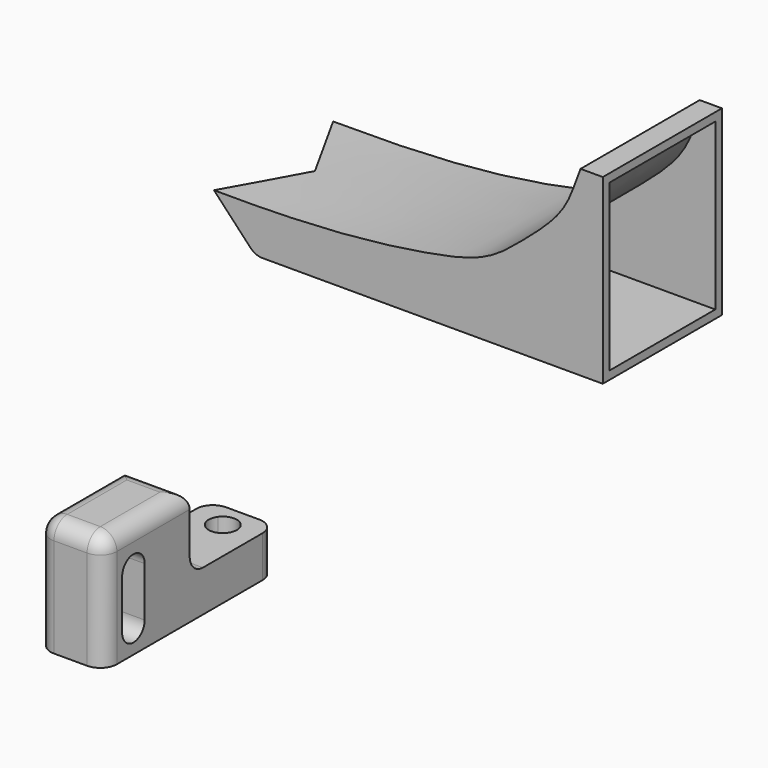
from build123d import *

# Parameters (mm, degrees)
F0_W      = 47
F0_H      = 18
F1_DEPTH  = 22
F4_DEPTH  = 25
F5_DEPTH  = 25
F7_T      = -1
F2_W      = 16
F2_H      = 20
F8_DEPTH  = 1
F9_W      = 8
F9_H      = 26
F10_DEPTH = 14
F11_W     = 13
F11_H     = 9
F12_DEPTH = 25
F13_R     = 2
F15_DEPTH = 25
F17_DEPTH = 25
F19_W     = 6.1407467425
F19_H     = 16
F20_DEPTH = 2
F21_R     = 2
F23_DEPTH = 16
F24_DEPTH = 25


# Not quite as in the source:
# - ends of sketch curves that miss each other by under 0.0002 mm in the source are joined


with BuildPart() as f1:
    # F0 (on Top) → F1 (new body)
    with BuildSketch(Plane.XY):
        with Locations((-23.5, 9)):
            Rectangle(F0_W, F0_H)
    extrude(amount=F1_DEPTH)

    # F3 (on face) → F4 (cut)
    with BuildSketch(Plane.XZ):
        with BuildLine():
            add(Edge.make_bspline(
                [(-2.6882688196, 22), (-3.2770454434, 20.6391466758), (-4.1784598757, 16.8748983141), (-9.4041486141, 12.3630724805), (-13.9335501605, 8.4565637973), (-23.0360767099, 6.5368633633), (-34.0870933489, 5.200595818), (-47, 5.3147859871)],
                knots=[0, 0, 0, 0, 0.1494824851, 0.3218138719, 0.4814084184, 0.6655862643, 1, 1, 1, 1], degree=3))
            Line((-2.6882688196, 22), (-47, 22))
            Line((-47, 22), (-47, 5.3147859871))
        make_face()
    extrude(amount=-F4_DEPTH, mode=Mode.SUBTRACT)

    # F3 (on face) → F5 (cut)
    with BuildSketch(Plane.XZ):
        Polygon((-42, 0), (-47, 5.3147859871), (-47, 0), align=None)
    extrude(amount=-F5_DEPTH, mode=Mode.SUBTRACT)

    # F7
    f7_openings = [f1.faces().sort_by_distance(p)[0] for p in [
        (-44.5, 9, 2.657393),
    ]]
    offset(amount=F7_T, openings=f7_openings, kind=Kind.INTERSECTION)

    # F2 (on face) → F8 (cut)
    with BuildSketch(Plane.YZ):
        with Locations((9, 11)):
            Rectangle(F2_W, F2_H)
    extrude(amount=-F8_DEPTH, mode=Mode.SUBTRACT)

    # F19 (on face) → F20 (cut)
    with BuildSketch(Plane(origin=(0, 0, 0), x_dir=(1, 0, 0), z_dir=(0, 0, -1))):
        with Locations((-38.9296266288, -9)):
            Rectangle(F19_W, F19_H)
        Polygon((-42, -1), (-42.6852083329, -1), (-43.1045070291, -1), (-43.1045070291, -17), (-42.6852083329, -17), (-42, -17), align=None)
    extrude(amount=-F20_DEPTH, mode=Mode.SUBTRACT)

    # F21
    f21_edges = [f1.edges().sort_by_distance(p)[0] for p in [
        (-35.859253, 17, 0.5),
        (-35.859253, 1, 0.5),
        (-42, 0.5, 0),
        (-42, 17.5, 0),
    ]]
    fillet(f21_edges, radius=F21_R)

    # F22 (on face) → F23 (join, through all)
    with BuildSketch(Plane.XZ.offset(-17)):
        with BuildLine():
            add(Edge.make_bspline(
                [(-45.979261035, 4.3077080456), (-45.9230921355, 4.3074304854), (-45.8669231813, 4.3071662313), (-45.8107541815, 4.3069151492), (-45.7545851445, 4.306677229), (-45.6984160781, 4.3064526573), (-45.6422469881, 4.3062418902), (-45.5860778784, 4.3060457258), (-44.541461727, 4.3026916555), (-43.5530151209, 4.3039144034), (-42.564580075, 4.309797802), (-41.5761785653, 4.3206346602), (-40.5878433409, 4.3367473036), (-39.599618044, 4.3584926715), (-38.61155733, 4.3862671393), (-37.6237268056, 4.4205065789)],
                knots=[0.1765693684, 0.1765693684, 0.1765693684, 0.1765693684, 0.1765693684, 0.1765693684, 0.1765693684, 0.1765693684, 0.1765693684, 0.1823209871, 0.1823209871, 0.1823209871, 0.1823209871, 0.1823209871, 0.1823209871, 0.1823209871, 0.2835362009, 0.2835362009, 0.2835362009, 0.2835362009, 0.2835362009, 0.2835362009, 0.2835362009, 0.2835362009, 0.2835362009], degree=8))
            Line((-45.979261035, 4.3077080456), (-44.6482196738, 2.8149441627))
            Line((-44.6482196738, 2.8149441627), (-37.6237268056, 4.4205065789))
        make_face()
    extrude(amount=F23_DEPTH)

    # F18 (on face) → F24 (cut)
    with BuildSketch(Plane(origin=(0, 0, 0), x_dir=(1, 0, 0), z_dir=(0, 0, -1))):
        Polygon((-47, -17.9847120319), (-46.9578729263, -17.9241712673), (-42, -9), (-47, 0), align=None)
    extrude(amount=-F24_DEPTH, mode=Mode.SUBTRACT)


with BuildPart() as f10:
    # F9 (on Top) → F10 (new body)
    with BuildSketch(Plane.XY):
        with Locations((-4, -62.4234300312)):
            Rectangle(F9_W, F9_H)
    extrude(amount=F10_DEPTH)

    # F11 (on face) → F12 (cut)
    with BuildSketch(Plane.YZ):
        with Locations((-55.9234300312, 9.5)):
            Rectangle(F11_W, F11_H)
    extrude(amount=-F12_DEPTH, mode=Mode.SUBTRACT)

    # F13
    f13_edges = [f10.edges().sort_by_distance(p)[0] for p in [
        (-4, -75.42343, 14),
        (-8, -75.42343, 7),
        (0, -75.42343, 7),
        (0, -68.92343, 14),
        (-8, -68.92343, 14),
        (-4, -62.42343, 5),
        (0, -49.42343, 2.5),
        (-8, -49.42343, 2.5),
        (-4, -62.42343, 14),
    ]]
    fillet(f13_edges, radius=F13_R)

    # F14 (on face) → F15 (cut)
    with BuildSketch(Plane.YZ):
        with BuildLine():
            ThreePointArc((-72.6234300312, 3), (-70.9234300312, 4.7), (-69.2234300312, 3))
            Line((-69.2234300312, 3), (-69.2234300312, 9))
            ThreePointArc((-69.2234300312, 9), (-70.9234300312, 7.3), (-72.6234300312, 9))
            Line((-72.6234300312, 9), (-72.6234300312, 3))
        make_face()
        with BuildLine():
            ThreePointArc((-72.6234300312, 9), (-70.9234300312, 7.3), (-69.2234300312, 9))
            ThreePointArc((-69.2234300312, 9), (-70.9234300312, 10.7), (-72.6234300312, 9))
        make_face()
        with BuildLine():
            ThreePointArc((-72.6234300312, 3), (-70.9234300312, 1.3), (-69.2234300312, 3))
            ThreePointArc((-69.2234300312, 3), (-70.9234300312, 4.7), (-72.6234300312, 3))
        make_face()
    extrude(amount=-F15_DEPTH, mode=Mode.SUBTRACT)

    # F16 (on face) → F17 (cut)
    with BuildSketch(Plane.XY.offset(5)):
        with BuildLine():
            Line((-2.6252272915, -51.4234300312), (-5.3747727085, -51.4234300312))
            ThreePointArc((-5.3747727085, -51.4234300312), (-4.5257786585, -54.0400799012), (-2.3, -52.4234300312))
            ThreePointArc((-2.3, -52.4234300312), (-2.38335013, -51.8976513726), (-2.6252272915, -51.4234300312))
        make_face()
        with BuildLine():
            ThreePointArc((-2.6252272915, -51.4234300312), (-4, -50.7234300312), (-5.3747727085, -51.4234300312))
            Line((-5.3747727085, -51.4234300312), (-2.6252272915, -51.4234300312))
        make_face()
    extrude(amount=-F17_DEPTH, mode=Mode.SUBTRACT)


solid = Compound([f1.part, f10.part])
